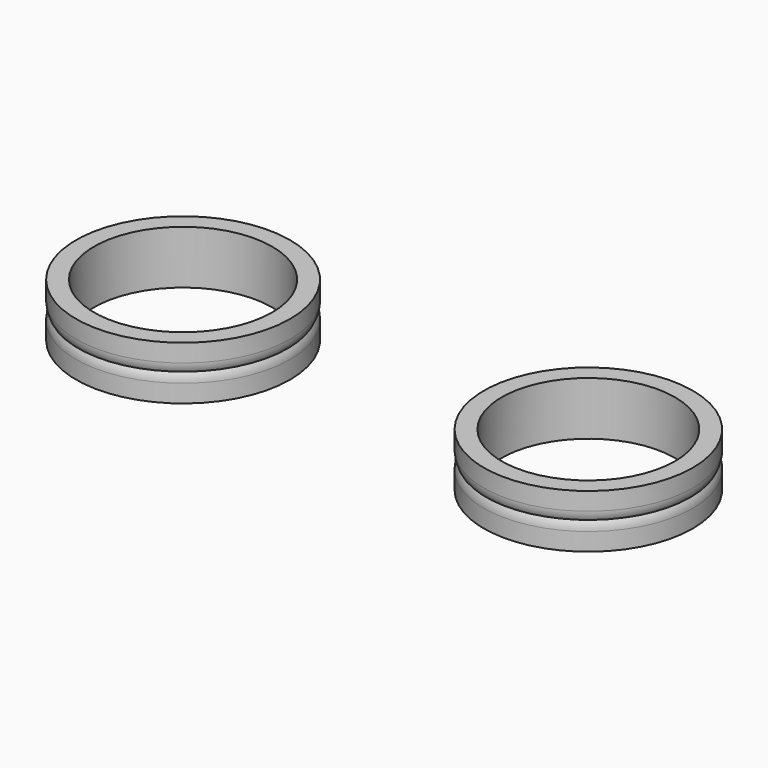
from build123d import *


with BuildPart() as f1:
    # F0 (on Front) → F1 (revolve)
    with BuildSketch(Plane.XZ):
        with BuildLine():
            Line((11.0075026751, 1.8), (11.0075026751, 0))
            ThreePointArc((11.0075026751, 0), (12.2802948812, 0.5272077939), (12.8075026751, 1.8))
            ThreePointArc((12.8075026751, 1.8), (12.7461691624, 2.2658742812), (12.5663484019, 2.7))
            ThreePointArc((12.5663484019, 2.7), (11.9075026751, 2.0411542732), (11.0075026751, 1.8))
        make_face()
        with BuildLine():
            ThreePointArc((12.8075026751, 1.8), (12.2802948812, 0.5272077939), (11.0075026751, 0))
            Line((11.0075026751, 0), (12.8075026751, 0))
            Line((12.8075026751, 0), (12.8075026751, 1.8))
        make_face()
        with BuildLine():
            Line((11.0075026751, 2.7), (11.0075026751, 1.8))
            ThreePointArc((11.0075026751, 1.8), (11.9075026751, 2.0411542732), (12.5663484019, 2.7))
            ThreePointArc((12.5663484019, 2.7), (12.528210521, 2.7630408337), (12.4875246825, 2.8244680851))
            ThreePointArc((12.4875246825, 2.8244680851), (11.8429538845, 3.3943717498), (11.0075026751, 3.6))
            Line((11.0075026751, 3.6), (11.0075026751, 2.7))
        make_face()
        with BuildLine():
            ThreePointArc((12.4875246825, 2.8244680851), (12.528210521, 2.7630408337), (12.5663484019, 2.7))
            ThreePointArc((12.5663484019, 2.7), (12.7461691624, 3.1341257188), (12.8075026751, 3.6))
            Line((12.8075026751, 3.6), (12.8075026751, 5.4))
            Line((12.8075026751, 5.4), (11.0075026751, 5.4))
            Line((11.0075026751, 5.4), (11.0075026751, 3.6))
            ThreePointArc((11.0075026751, 3.6), (11.8429538845, 3.3943717498), (12.4875246825, 2.8244680851))
        make_face()
    revolve(axis=Axis((2.0075026751, 0, 2.4673056323), (0, 0, -1)))


with BuildPart() as f3:
    # F2 (on Front) → F3 (revolve)
    with BuildSketch(Plane.XZ):
        with BuildLine():
            Line((53.4780735552, 5.4), (51.6780735552, 5.4))
            Line((51.6780735552, 5.4), (51.6780735552, 3.6))
            ThreePointArc((51.6780735552, 3.6), (52.5780735552, 3.3588457268), (53.236919282, 2.7))
            ThreePointArc((53.236919282, 2.7), (53.4167400426, 3.1341257188), (53.4780735552, 3.6))
            Line((53.4780735552, 3.6), (53.4780735552, 5.4))
        make_face()
        with BuildLine():
            ThreePointArc((53.236919282, 2.7), (52.5780735552, 3.3588457268), (51.6780735552, 3.6))
            Line((51.6780735552, 3.6), (51.6780735552, 1.8))
            ThreePointArc((51.6780735552, 1.8), (52.5780735552, 2.0411542732), (53.236919282, 2.7))
        make_face()
        with BuildLine():
            ThreePointArc((53.236919282, 2.7), (52.5780735552, 2.0411542732), (51.6780735552, 1.8))
            Line((51.6780735552, 1.8), (51.6780735552, 0))
            Line((51.6780735552, 0), (53.4780735552, 0))
            Line((53.4780735552, 0), (53.4780735552, 1.8))
            ThreePointArc((53.4780735552, 1.8), (53.4167400426, 2.2658742812), (53.236919282, 2.7))
        make_face()
    revolve(axis=Axis((42.9280735552, 0, 5.6644450251), (0, 0, 1)))


solid = Compound([f1.part, f3.part])
